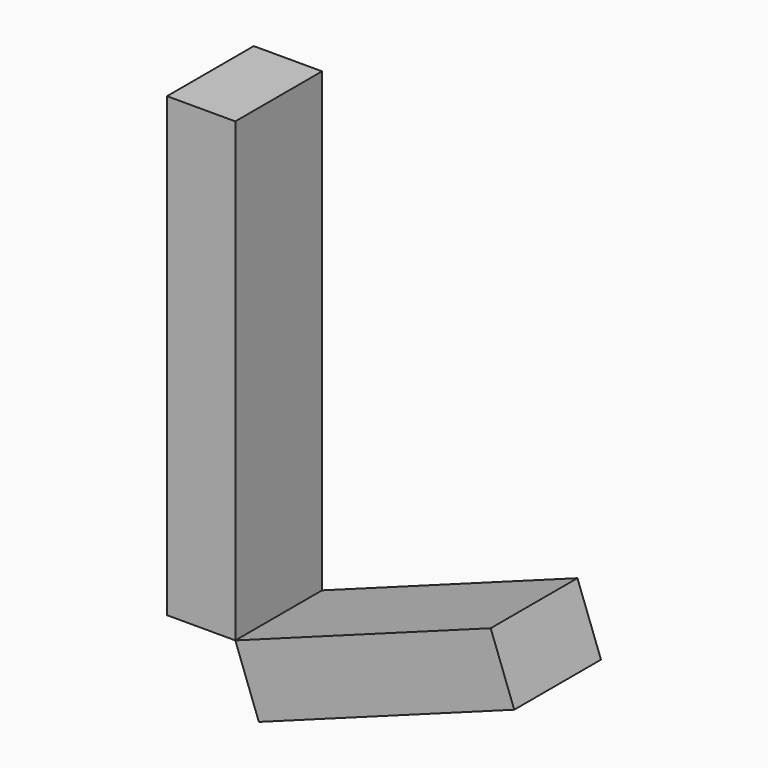
from build123d import *

# Parameters (mm, degrees)
F1_E1_W  = 101.2163225714
F1_E1_H  = 40.3352081776
F2_DEPTH = 25.4
F1_E0_W  = 169.9852496386
F1_E0_H  = 40.3352081776
F3_DEPTH = 25.4


with BuildPart() as f2:
    # F1_E1 (on explicit) → F2 (new body)
    with BuildSketch(Plane(origin=(-57.5071722269, 0, -75.5722895265), x_dir=(0.9387011168, 0, 0.3447320893), z_dir=(0.3447320893, 0, -0.9387011168))):
        with Locations((50.6081612857, 20.1676040888)):
            Rectangle(F1_E1_W, F1_E1_H)
    extrude(amount=F2_DEPTH)


with BuildPart() as f3:
    # F1_E0 (on explicit) → F3 (new body)
    with BuildSketch(Plane(origin=(-57.5071722269, 0, 94.4129601121), x_dir=(0, 0, -1), z_dir=(-1, 0, 0))):
        with Locations((84.9926248193, 20.1676040888)):
            Rectangle(F1_E0_W, F1_E0_H)
    extrude(amount=F3_DEPTH)


solid = Compound([f2.part, f3.part])
